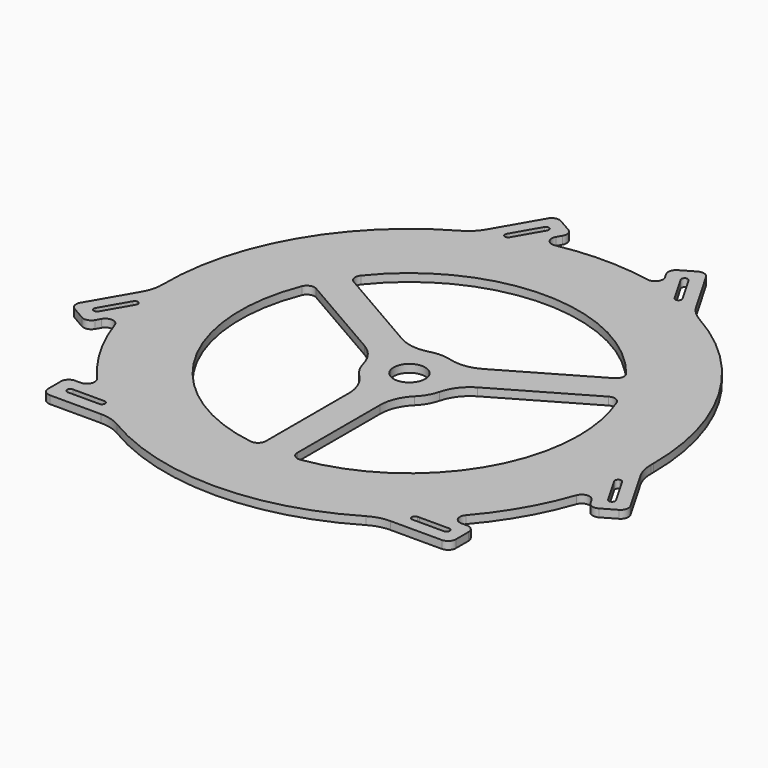
from build123d import *

# Parameters (mm, degrees)
F0_R     = 10
F1_DEPTH = 5
F2_R     = 5
F3_R     = 5
F4_R     = 25
F5_R     = 25
F6_R     = 5


# Not quite as in the source:
# - ends of sketch curves that miss each other by under 0.0002 mm in the source are joined


with BuildPart() as f1:
    # F0 (on Top) → F1 (new body)
    with BuildSketch(Plane.XY):
        with BuildLine():
            ThreePointArc((154.7685858954, -8.4666888412), (154.9421356729, -4.2349253955), (155, 0))
            ThreePointArc((155, 0), (132.0663621555, 81.1386220428), (70.0519227484, 138.2668728194))
            ThreePointArc((70.0519227484, 138.2668728194), (62.8960752724, 141.6653934994), (55.5759359282, 144.6938676852))
            ThreePointArc((55.5759359282, 144.6938676852), (53.8706420703, 143.993176318), (52.3166727987, 144.9852322827))
            Line((52.3166727987, 144.9852322827), (51.6490211362, 146.1416388839))
            ThreePointArc((51.6490211362, 146.1416388839), (46.0520817915, 148.0006951425), (40.3884712615, 149.6454856959))
            ThreePointArc((40.3884712615, 149.6454856959), (2.3057e-06, 155), (-40.3884668093, 149.6454868975))
            ThreePointArc((-40.3884668093, 149.6454868975), (-46.0520770675, 148.0006966124), (-51.6490161547, 146.1416406444))
            Line((-51.6490161547, 146.1416406445), (-52.3166688853, 144.9852321932))
            ThreePointArc((-52.3166688853, 144.9852321932), (-53.8706389409, 143.9931761584), (-55.5759330313, 144.6938687979))
            ThreePointArc((-55.5759330313, 144.6938687979), (-62.8960721537, 141.665394884), (-70.0519194288, 138.2668745012))
            ThreePointArc((-70.0519194288, 138.2668745012), (-134.2339375866, 77.5), (-154.7685855343, -8.4666954414))
            ThreePointArc((-154.7685855343, -8.4666954414), (-154.1338668835, -16.3631011587), (-153.0965326665, -24.2167645548))
            ThreePointArc((-153.0965326665, -24.2167645548), (-151.9167610651, -24.9023775772), (-151.4512795032, -26.1850518006))
            ThreePointArc((-151.4512795032, -26.1850518006), (-151.5194278506, -26.7026898908), (-151.7192286956, -27.1850518006))
            Line((-151.7192286956, -27.1850518006), (-152.3868814262, -28.3414602518))
            ThreePointArc((-152.3868814262, -28.3414602518), (-151.1984015779, -34.1180796687), (-149.7910266196, -39.845305172))
            ThreePointArc((-149.7910266196, -39.845305172), (-134.2339373892, -77.500000342), (-109.4025592509, -109.8001822829))
            ThreePointArc((-109.4025592509, -109.8001822829), (-105.1463222254, -113.8826190535), (-100.7378611443, -117.800183922))
            Line((-100.7378611443, -117.8001839221), (-99.4025592509, -117.8001839221))
            ThreePointArc((-99.4025592509, -117.8001839221), (-97.9883456885, -118.3859703597), (-97.4025592509, -119.8001839221))
            ThreePointArc((-97.4025592509, -119.8001839221), (-97.4322899717, -120.143751918), (-97.5205982187, -120.4771053897))
            ThreePointArc((-97.5205982187, -120.4771053897), (-91.2377891853, -125.3022977626), (-84.7166561444, -129.8001855612))
            ThreePointArc((-84.7166561444, -129.8001855612), (0, -155), (84.7166561444, -129.8001855612))
            ThreePointArc((84.7166561444, -129.8001855612), (91.2377891853, -125.3022977626), (97.5205982187, -120.4771053897))
            ThreePointArc((97.5205982187, -120.4771053897), (97.7664292231, -118.6499324137), (99.4025592509, -117.8001839221))
            Line((99.4025592509, -117.8001839221), (100.7378611443, -117.8001839221))
            ThreePointArc((100.7378611443, -117.800183922), (105.1463222254, -113.8826190535), (109.4025592509, -109.8001822829))
            ThreePointArc((109.4025592509, -109.8001822829), (134.233938542, -77.4999983451), (149.791027805, -39.8453007155))
            ThreePointArc((149.791027805, -39.8453007155), (151.1984026669, -34.1180748426), (152.3868823923, -28.3414550574))
            Line((152.3868823923, -28.3414550574), (151.719230036, -27.1850472546))
            ThreePointArc((151.719230036, -27.1850472546), (151.6370691989, -25.3432419871), (153.0965333673, -24.2167601241))
            ThreePointArc((153.0965333673, -24.2167601241), (154.1338674692, -16.3630956418), (154.7685858954, -8.4666888412))
        make_face()
        with BuildLine():
            Line((100.0897495333, 46.2398384524), (97.6940532073, 44.8566825337))
            ThreePointArc((97.6940532073, 44.8566825337), (105.019904589, 22.9579973017), (107.5, 0))
            ThreePointArc((107.5, 0), (79.4709066263, -72.3921611779), (10, -107.033873143))
            Line((10, -107.033873143), (10, -109.8001822829))
            Line((10, -109.8001822829), (0, -109.8001822829))
            Line((0, -109.8001822829), (-10, -109.8001822829))
            Line((-10, -109.8001822829), (-10, -107.033873143))
            ThreePointArc((-10, -107.033873143), (-93.0977309068, -53.75), (-97.6940532073, 44.8566825337))
            Line((-97.6940532073, 44.8566825337), (-100.0897467145, 46.2398368249))
            Line((-100.0897467145, 46.2398368249), (-90.0897467145, 63.5603449006))
            Line((-90.0897467145, 63.5603449006), (-87.6940532073, 62.1771906094))
            ThreePointArc((-87.6940532073, 62.1771906094), (0, 107.5), (87.6940532073, 62.1771906094))
            Line((87.6940532073, 62.1771906094), (90.0897495333, 63.5603465281))
            Line((90.0897495333, 63.5603465281), (100.0897495333, 46.2398384524))
        make_face(mode=Mode.SUBTRACT)
        with BuildLine():
            ThreePointArc((55.5759359282, 144.6938676852), (62.8960752724, 141.6653934994), (70.0519227484, 138.2668728194))
            Line((70.0519227484, 138.2668728194), (47.7089766448, 176.9659938193))
            Line((47.7089766448, 176.9659938193), (30.3884705677, 166.9659949732))
            Line((30.3884705677, 166.9659949732), (40.3884712615, 149.6454856959))
            ThreePointArc((40.3884712615, 149.6454856959), (46.0520817915, 148.0006951425), (51.6490211362, 146.1416388839))
            Line((51.6490211362, 146.1416388839), (42.3166727987, 162.3057403584))
            ThreePointArc((42.3166727987, 162.3057403584), (43.0487236063, 165.037791166), (45.7807744138, 164.3057403584))
            Line((45.7807744138, 164.3057403584), (55.7807744138, 146.9852322827))
            ThreePointArc((55.7807744138, 146.9852322827), (55.9805752588, 146.5028703729), (56.0487236063, 145.9852322827))
            ThreePointArc((56.0487236063, 145.9852322827), (55.9268110169, 145.2976367053), (55.5759359282, 144.6938676852))
        make_face()
        with BuildLine():
            Line((177.1115338821, -47.1658099451), (154.7685858954, -8.4666888412))
            ThreePointArc((154.7685858954, -8.4666888412), (154.1338674692, -16.3630956418), (153.0965333673, -24.2167601241))
            ThreePointArc((153.0965333673, -24.2167601241), (154.2930861111, -24.3708356099), (155.1833316512, -25.1850472546))
            Line((155.1833316512, -25.1850472546), (165.1833316512, -42.5055553303))
            ThreePointArc((165.1833316512, -42.5055553303), (165.3831324962, -42.9879172401), (165.4512808436, -43.5055553303))
            ThreePointArc((165.4512808436, -43.5055553303), (163.9689189338, -45.4374069829), (161.719230036, -44.5055553303))
            Line((161.719230036, -44.5055553303), (152.3868823923, -28.3414550574))
            ThreePointArc((152.3868823923, -28.3414550574), (151.1984026669, -34.1180748426), (149.791027805, -39.8453007155))
            Line((149.791027805, -39.8453007155), (159.791027805, -57.1658087912))
            Line((159.791027805, -57.1658087912), (177.1115338821, -47.1658099451))
        make_face()
        with BuildLine():
            ThreePointArc((-51.6490161547, 146.1416406444), (-46.0520770675, 148.0006966124), (-40.3884668093, 149.6454868975))
            Line((-40.3884668093, 149.6454868975), (-30.3884668093, 166.9659949732))
            Line((-30.3884668093, 166.9659949732), (-47.7089725764, 176.9659936403))
            Line((-47.7089725764, 176.9659936403), (-70.0519194288, 138.2668745012))
            ThreePointArc((-70.0519194288, 138.2668745012), (-62.8960721537, 141.665394884), (-55.5759330313, 144.6938687979))
            ThreePointArc((-55.5759330313, 144.6938687979), (-56.0407757277, 145.8071514412), (-55.7807705004, 146.9852321932))
            Line((-55.7807705004, 146.9852321932), (-45.7807705004, 164.3057402689))
            ThreePointArc((-45.7807705004, 164.3057402689), (-43.5310816027, 165.2375919215), (-42.0487196929, 163.3057402689))
            ThreePointArc((-42.0487196929, 163.3057402689), (-42.1168680403, 162.7881021787), (-42.3166688853, 162.3057402689))
            Line((-42.3166688853, 162.3057402689), (-51.6490161547, 146.1416406445))
        make_face()
        with BuildLine():
            Line((129.4025592509, -109.8001822829), (109.4025592509, -109.8001822829))
            ThreePointArc((109.4025592509, -109.8001822829), (105.1463222254, -113.8826190535), (100.7378611443, -117.800183922))
            Line((100.7378611443, -117.800183922), (119.4025592509, -117.8001839221))
            ThreePointArc((119.4025592509, -117.8001839221), (120.8167728132, -118.3859703597), (121.4025592509, -119.8001839221))
            ThreePointArc((121.4025592509, -119.8001839221), (120.8167728132, -121.2143974844), (119.4025592509, -121.8001839221))
            Line((119.4025592509, -121.8001839221), (99.4025592509, -121.8001842499))
            ThreePointArc((99.4025592509, -121.8001842499), (98.2523077425, -121.4363139498), (97.5205982187, -120.4771053897))
            ThreePointArc((97.5205982187, -120.4771053897), (91.2377891853, -125.3022977626), (84.7166561444, -129.8001855612))
            Line((84.7166561444, -129.8001855612), (129.4025592509, -129.8001855612))
            Line((129.4025592509, -129.8001855612), (129.4025592509, -109.8001822829))
        make_face()
        with BuildLine():
            ThreePointArc((-153.0965326665, -24.2167645548), (-154.1338668835, -16.3631011587), (-154.7685855343, -8.4666954414))
            Line((-154.7685855343, -8.4666954414), (-177.1115323867, -47.1658145805))
            Line((-177.1115323867, -47.1658145805), (-159.7910266196, -57.1658132477))
            Line((-159.7910266196, -57.1658132477), (-149.7910266196, -39.845305172))
            ThreePointArc((-149.7910266196, -39.845305172), (-151.1984015779, -34.1180796687), (-152.3868814262, -28.3414602518))
            Line((-152.3868814262, -28.3414602518), (-161.7192286956, -44.5055598762))
            ThreePointArc((-161.7192286956, -44.5055598762), (-164.4512795031, -45.2376106838), (-165.1833303107, -42.5055598762))
            Line((-165.1833303107, -42.5055598762), (-155.1833303107, -25.1850518006))
            ThreePointArc((-155.1833303107, -25.1850518006), (-154.2930850654, -24.3708402927), (-153.0965326665, -24.2167645548))
        make_face()
        with BuildLine():
            Line((-129.4025592509, -129.8001855612), (-84.7166561444, -129.8001855612))
            ThreePointArc((-84.7166561444, -129.8001855612), (-91.2377891853, -125.3022977626), (-97.5205982187, -120.4771053897))
            ThreePointArc((-97.5205982187, -120.4771053897), (-98.2523077425, -121.4363139498), (-99.4025592509, -121.8001839221))
            Line((-99.4025592509, -121.8001839221), (-119.4025592509, -121.8001839221))
            ThreePointArc((-119.4025592509, -121.8001839221), (-121.4025592509, -119.8001839221), (-119.4025592509, -117.8001839221))
            Line((-119.4025592509, -117.8001839221), (-100.7378611443, -117.8001839221))
            ThreePointArc((-100.7378611443, -117.800183922), (-105.1463222254, -113.8826190535), (-109.4025592509, -109.8001822829))
            Line((-109.4025592509, -109.8001822829), (-129.4025592509, -109.8001822829))
            Line((-129.4025592509, -109.8001822829), (-129.4025592509, -129.8001855612))
        make_face()
        with BuildLine():
            ThreePointArc((10, -22.9128784748), (20.9165006634, -13.6930639376), (25, 0))
            ThreePointArc((25, 0), (24.9607529016, 1.400290894), (24.843134833, 2.7961851995))
            ThreePointArc((24.843134833, 2.7961851995), (21.6506350946, 12.5), (14.843134833, 20.1166932752))
            ThreePointArc((14.843134833, 20.1166932752), (0, 25), (-14.843134833, 20.1166932752))
            ThreePointArc((-14.843134833, 20.1166932752), (-21.6506350946, 12.5), (-24.843134833, 2.7961851995))
            ThreePointArc((-24.843134833, 2.7961851995), (-21.6506350946, -12.5), (-10, -22.9128784748))
            ThreePointArc((-10, -22.9128784748), (0, -25), (10, -22.9128784748))
        make_face()
        Circle(F0_R, mode=Mode.SUBTRACT)
        with BuildLine():
            ThreePointArc((14.843134833, 20.1166932752), (21.6506350946, 12.5), (24.843134833, 2.7961851995))
            Line((24.843134833, 2.7961851995), (97.6940532073, 44.8566825337))
            ThreePointArc((97.6940532073, 44.8566825337), (93.0977309068, 53.75), (87.6940532073, 62.1771906094))
            Line((87.6940532073, 62.1771906094), (14.843134833, 20.1166932752))
        make_face()
        with BuildLine():
            Line((10, -107.033873143), (10, -22.9128784748))
            ThreePointArc((10, -22.9128784748), (0, -25), (-10, -22.9128784748))
            Line((-10, -22.9128784748), (-10, -107.033873143))
            ThreePointArc((-10, -107.033873143), (0, -107.5), (10, -107.033873143))
        make_face()
        with BuildLine():
            ThreePointArc((87.6940532073, 62.1771906094), (93.0977309068, 53.75), (97.6940532073, 44.8566825337))
            Line((97.6940532073, 44.8566825337), (100.0897495333, 46.2398384524))
            Line((100.0897495333, 46.2398384524), (90.0897495333, 63.5603465281))
            Line((90.0897495333, 63.5603465281), (87.6940532073, 62.1771906094))
        make_face()
        with BuildLine():
            Line((10, -109.8001822829), (10, -107.033873143))
            ThreePointArc((10, -107.033873143), (0, -107.5), (-10, -107.033873143))
            Line((-10, -107.033873143), (-10, -109.8001822829))
            Line((-10, -109.8001822829), (0, -109.8001822829))
            Line((0, -109.8001822829), (10, -109.8001822829))
        make_face()
        with BuildLine():
            ThreePointArc((-24.843134833, 2.7961851995), (-21.6506350946, 12.5), (-14.843134833, 20.1166932752))
            Line((-14.843134833, 20.1166932752), (-87.6940532073, 62.1771906094))
            ThreePointArc((-87.6940532073, 62.1771906094), (-93.0977309068, 53.75), (-97.6940532073, 44.8566825337))
            Line((-97.6940532073, 44.8566825337), (-24.843134833, 2.7961851995))
        make_face()
        with BuildLine():
            ThreePointArc((-97.6940532073, 44.8566825337), (-93.0977309068, 53.75), (-87.6940532073, 62.1771906094))
            Line((-87.6940532073, 62.1771906094), (-90.0897467145, 63.5603449006))
            Line((-90.0897467145, 63.5603449006), (-100.0897467145, 46.2398368249))
            Line((-100.0897467145, 46.2398368249), (-97.6940532073, 44.8566825337))
        make_face()
    extrude(amount=F1_DEPTH)

    # F2
    f2_edges = [f1.edges().sort_by_distance(p)[0] for p in [
        (-47.708973, 176.965994, 2.5),
        (-30.388467, 166.965995, 2.5),
        (30.388471, 166.965995, 2.5),
        (47.708977, 176.965994, 2.5),
        (177.111534, -47.16581, 2.5),
        (-177.111532, -47.165815, 2.5),
        (-129.402559, -109.800182, 2.5),
        (129.402559, -109.800182, 2.5),
        (159.791028, -57.165809, 2.5),
        (129.402559, -129.800186, 2.5),
        (-129.402559, -129.800186, 2.5),
        (-159.791027, -57.165813, 2.5),
    ]]
    fillet(f2_edges, radius=F2_R)

    # F3
    f3_edges = [f1.edges().sort_by_distance(p)[0] for p in [
        (-149.791027, -39.845305, 2.5),
        (149.791028, -39.845301, 2.5),
        (40.388471, 149.645486, 2.5),
        (-40.388467, 149.645487, 2.5),
        (-109.402559, -109.800182, 2.5),
        (109.402559, -109.800182, 2.5),
    ]]
    fillet(f3_edges, radius=F3_R)

    # F4
    f4_edges = [f1.edges().sort_by_distance(p)[0] for p in [
        (-70.051919, 138.266875, 2.5),
        (-154.768586, -8.466695, 2.5),
        (70.051923, 138.266873, 2.5),
        (154.768586, -8.466689, 2.5),
        (-84.716656, -129.800186, 2.5),
        (84.716656, -129.800186, 2.5),
    ]]
    fillet(f4_edges, radius=F4_R)

    # F5
    f5_edges = [f1.edges().sort_by_distance(p)[0] for p in [
        (-10, -22.912878, 2.5),
        (-24.843135, 2.796185, 2.5),
        (10, -22.912878, 2.5),
        (24.843135, 2.796185, 2.5),
        (14.843135, 20.116693, 2.5),
        (-14.843135, 20.116693, 2.5),
    ]]
    fillet(f5_edges, radius=F5_R)

    # F6
    f6_edges = [f1.edges().sort_by_distance(p)[0] for p in [
        (-97.694053, 44.856683, 2.5),
        (97.694053, 44.856683, 2.5),
        (10, -107.033873, 2.5),
        (-87.694053, 62.177191, 2.5),
        (87.694053, 62.177191, 2.5),
        (-10, -107.033873, 2.5),
    ]]
    fillet(f6_edges, radius=F6_R)


solid = f1.part
